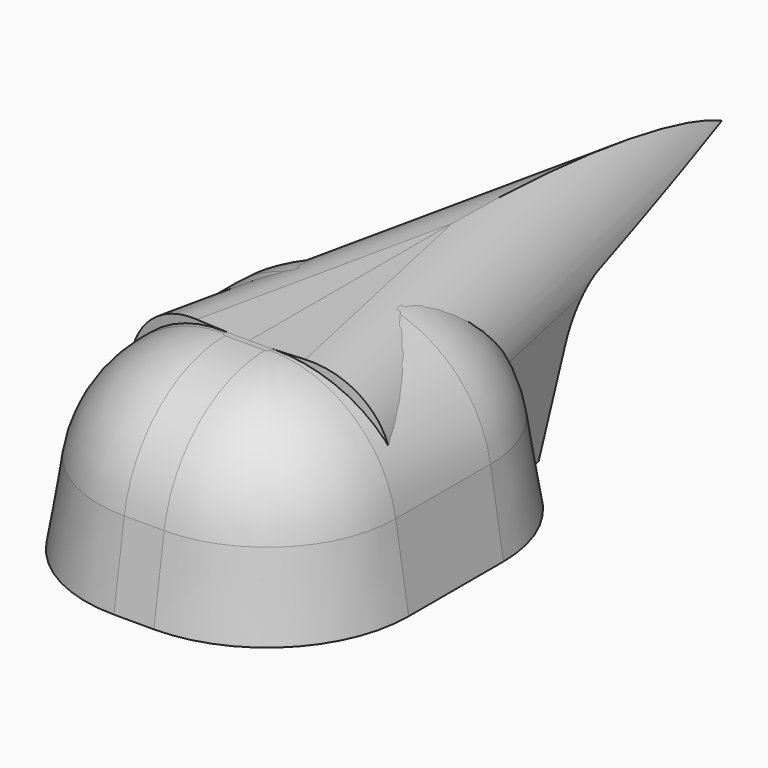
from build123d import *

# Parameters (mm, degrees)
F2_DEPTH    = 169.672
F2_TAPER    = 9
F3_R        = 114.3
F6_ANGLE    = 12.1829310863
F7_T2_ANGLE = 12.1829310863
F7_T6_DEPTH = 901.8811791581
F7_S7_R     = 558.1432208419
F7_T8_DEPTH = 470


# Not quite as in the source:
# - a fillet or chamfer that OpenCascade refuses, or shapes differently, is made with other operations: its cross-section is extruded or revolved along the edge and cut away or added


with BuildPart() as f2:
    # F1 (on offset) → F2 (new body)
    with BuildSketch(Plane.XY.offset(56.896)):
        with BuildLine():
            ThreePointArc((-144.9196487665, -53.105003047), (-107.7222099772, -142.9075642577), (-17.9196487665, -180.105003047))
            Line((-17.9196487665, -180.105003047), (0, -180.105003047))
            Line((0, -180.105003047), (17.9196487665, -180.105003047))
            ThreePointArc((17.9196487665, -180.105003047), (107.7222099772, -142.9075642577), (144.9196487665, -53.105003047))
            Line((144.9196487665, -53.105003047), (144.9196487665, 0))
            Line((144.9196487665, 0), (144.9196487665, 53.105003047))
            ThreePointArc((144.9196487665, 53.105003047), (107.7222099772, 142.9075642577), (17.9196487665, 180.105003047))
            Line((17.9196487665, 180.105003047), (0, 180.105003047))
            Line((0, 180.105003047), (-17.9196487665, 180.105003047))
            ThreePointArc((-17.9196487665, 180.105003047), (-107.7222099772, 142.9075642577), (-144.9196487665, 53.105003047))
            Line((-144.9196487665, 53.105003047), (-144.9196487665, 0))
            Line((-144.9196487665, 0), (-144.9196487665, -53.105003047))
        make_face()
    extrude(amount=F2_DEPTH, taper=F2_TAPER)

    # F3
    f3_edges = [f2.edges().sort_by_distance(p)[0] for p in [
        (-118.046244, 0, 226.568),
    ]]
    fillet(f3_edges, radius=F3_R)


with BuildPart() as f6:
    # F4 (on Right) → F6 (revolve)
    with BuildSketch(Plane.YZ):
        Polygon((-50.7769212127, 226.568), (-50.7769212127, 141.7786058209), (-50.7769212127, 56.896), (180.0686866045, 56.896), (239.6881223982, 160.0008904934), (505.895614624, 187.6315176487), (501.8542579455, 226.568), align=None)
    revolve(axis=Axis((0, 507.3662996292, 211.7486968637), (0, 0, -1)), revolution_arc=F6_ANGLE)

    # F7: fillet of radius 69.85 on 2 edges, made by hand

    # F7_s1 → F7_t2 (revolve)
    with BuildSketch(Plane.YZ):
        with BuildLine():
            ThreePointArc((221.8585221218, 129.1666673988), (244.3415795247, 152.8197661139), (275.1158289732, 163.6780587923))
            Line((275.1158289732, 163.6780587923), (274.9716041433, 165.0675940378))
            Line((274.9716041433, 165.0675940378), (238.8353434367, 161.3168823729))
            Line((238.8353434367, 161.3168823729), (220.6491511548, 129.8659748164))
            Line((220.6491511548, 129.8659748164), (221.8585221218, 129.1666673988))
        make_face()
    revolve(axis=Axis((0, 507.3662996292, 160.0008904934), (0, 0, -1)), revolution_arc=F7_T2_ANGLE)


with BuildPart() as f7_tool4:
    # F7_s5 → F7_t6 (new body)
    with BuildSketch(Plane(origin=(140.3484830453, 650.074981269, 0), x_dir=(0, 0, 1), z_dir=(-0.2110336063, -0.9774788064, 0))):
        with BuildLine():
            ThreePointArc((226.568, 37.2213399469), (206.1094086659, 86.6127486127), (156.718, 107.0713399469))
            Line((156.718, 107.0713399469), (156.718, 108.4683399469))
            Line((156.718, 108.4683399469), (227.965, 108.4683399469))
            Line((227.965, 108.4683399469), (227.965, 37.2213399469))
            Line((227.965, 37.2213399469), (226.568, 37.2213399469))
        make_face()
    extrude(amount=F7_T6_DEPTH)

    # F7_s7 → F7_t8 (intersect, symmetric)
    with BuildSketch(Plane.XY.offset(192.3)):
        with Locations((0, 507.3662996292)):
            Circle(F7_S7_R)
    extrude(amount=F7_T8_DEPTH, both=True, mode=Mode.INTERSECT)


with BuildPart() as f6_1:
    add(f6.part)

    # F7_t3: cut F7_tool4
    add(f7_tool4.part, mode=Mode.SUBTRACT)


with BuildPart() as f8_1:
    # F8: instance of F6
    add(f6_1.part.mirror(Plane.YZ))


solid = Compound([f2.part, f6_1.part, f8_1.part])
